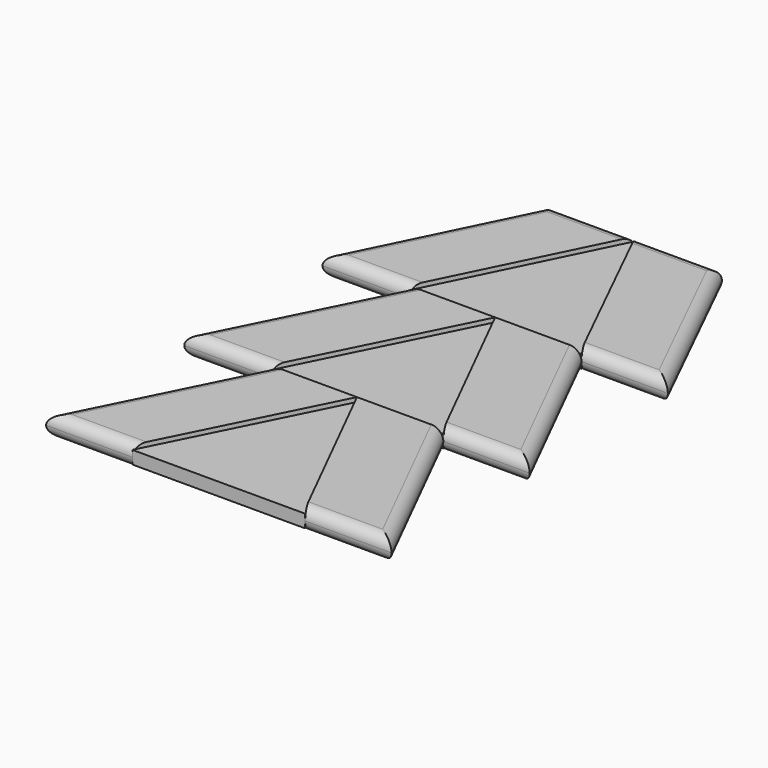
from build123d import *

# Parameters (mm, degrees)
F1_DEPTH = 3.175
F2_DEPTH = 1.905
F3_R     = 3.17499
F3_2_R   = 3.17499
F3_3_R   = 3.17499
F3_4_R   = 3.17499
F3_5_R   = 3.17499
F3_6_R   = 3.17499


# Not quite as in the source:
# - a fillet or chamfer is up to 0.001 mm smaller than in the source, because OpenCascade refuses the exact size


with BuildPart() as f1:
    # F0 (on Top) → F1 (new body, symmetric)
    with BuildSketch(Plane.XY):
        Polygon((0, 101.6), (25.4, 101.6), (50.8, 153.2299369574), (25.4, 153.2299369574), align=None)
    extrude(amount=F1_DEPTH, both=True)

    # F3#3 (radius 3.175 in the source; OpenCascade refuses exactly that, so slightly less here)
    f3_3_edges = [f1.edges().sort_by_distance(p)[0] for p in [
        (12.7, 127.414968, 3.175),
        (12.7, 127.414968, -3.175),
        (38.1, 153.229937, -3.175),
        (38.1, 153.229937, 3.175),
        (12.7, 101.6, 3.175),
        (12.7, 101.6, -3.175),
    ]]
    fillet(f3_3_edges, radius=F3_3_R)


with BuildPart() as f1b:
    # F0 (on Top) → F1, piece 2 (new body, symmetric)
    with BuildSketch(Plane.XY):
        Polygon((50.8, 153.2299369574), (76.2, 101.6), (101.6, 101.6), (76.2, 153.2299369574), align=None)
    extrude(amount=F1_DEPTH, both=True)

    # F3#4 (radius 3.175 in the source; OpenCascade refuses exactly that, so slightly less here)
    f3_4_edges = [f1b.edges().sort_by_distance(p)[0] for p in [
        (88.9, 127.414968, 3.175),
        (88.9, 127.414968, -3.175),
        (63.5, 153.229937, 3.175),
        (63.5, 153.229937, -3.175),
        (88.9, 101.6, 3.175),
        (88.9, 101.6, -3.175),
    ]]
    fillet(f3_4_edges, radius=F3_4_R)


with BuildPart() as f1c:
    # F0 (on Top) → F1, piece 3 (new body, symmetric)
    with BuildSketch(Plane.XY):
        Polygon((76.2, 101.6), (50.8, 101.6), (76.2, 50.8), (101.6, 50.8), align=None)
    extrude(amount=F1_DEPTH, both=True)

    # F3#5 (radius 3.175 in the source; OpenCascade refuses exactly that, so slightly less here)
    f3_5_edges = [f1c.edges().sort_by_distance(p)[0] for p in [
        (88.9, 76.2, 3.175),
        (88.9, 76.2, -3.175),
        (88.9, 50.8, -3.175),
        (88.9, 50.8, 3.175),
    ]]
    fillet(f3_5_edges, radius=F3_5_R)


with BuildPart() as f1d:
    # F0 (on Top) → F1, piece 4 (new body, symmetric)
    with BuildSketch(Plane.XY):
        Polygon((0, 50.8), (25.4, 50.8), (50.8, 101.6), (25.4, 101.6), align=None)
    extrude(amount=F1_DEPTH, both=True)

    # F3#2 (radius 3.175 in the source; OpenCascade refuses exactly that, so slightly less here)
    f3_2_edges = [f1d.edges().sort_by_distance(p)[0] for p in [
        (12.7, 76.2, 3.175),
        (12.7, 76.2, -3.175),
        (12.7, 50.8, 3.175),
        (12.7, 50.8, -3.175),
    ]]
    fillet(f3_2_edges, radius=F3_2_R)


with BuildPart() as f1e:
    # F0 (on Top) → F1, piece 5 (new body, symmetric)
    with BuildSketch(Plane.XY):
        Polygon((25.4, 50.8), (0, 0), (25.4, 0), (50.8, 50.8), align=None)
    extrude(amount=F1_DEPTH, both=True)

    # F3 (radius 3.175 in the source; OpenCascade refuses exactly that, so slightly less here)
    f3_edges = [f1e.edges().sort_by_distance(p)[0] for p in [
        (12.7, 25.4, 3.175),
        (12.7, 25.4, -3.175),
        (12.7, 0, 3.175),
        (12.7, 0, -3.175),
    ]]
    fillet(f3_edges, radius=F3_R)


with BuildPart() as f1f:
    # F0 (on Top) → F1, piece 6 (new body, symmetric)
    with BuildSketch(Plane.XY):
        Polygon((76.2, 50.8), (50.8, 50.8), (76.2, 0), (101.6, 0), align=None)
    extrude(amount=F1_DEPTH, both=True)

    # F3#6 (radius 3.175 in the source; OpenCascade refuses exactly that, so slightly less here)
    f3_6_edges = [f1f.edges().sort_by_distance(p)[0] for p in [
        (88.9, 25.4, 3.175),
        (88.9, 25.4, -3.175),
        (88.9, 0, 3.175),
        (88.9, 0, -3.175),
    ]]
    fillet(f3_6_edges, radius=F3_6_R)


with BuildPart() as f2:
    # F0 (on Top) → F2 (new body, symmetric)
    with BuildSketch(Plane.XY):
        Polygon((25.4, 101.6), (50.8, 101.6), (76.2, 101.6), (50.8, 153.2299369574), align=None)
    extrude(amount=F2_DEPTH, both=True)


with BuildPart() as f2b:
    # F0 (on Top) → F2, piece 2 (new body, symmetric)
    with BuildSketch(Plane.XY):
        Polygon((50.8, 101.6), (25.4, 50.8), (50.8, 50.8), (76.2, 50.8), align=None)
    extrude(amount=F2_DEPTH, both=True)


with BuildPart() as f2c:
    # F0 (on Top) → F2, piece 3 (new body, symmetric)
    with BuildSketch(Plane.XY):
        Polygon((50.8, 50.8), (25.4, 0), (76.2, 0), align=None)
    extrude(amount=F2_DEPTH, both=True)


solid = Compound([f1.part, f1b.part, f1c.part, f1d.part, f1e.part, f1f.part, f2.part, f2b.part, f2c.part])
